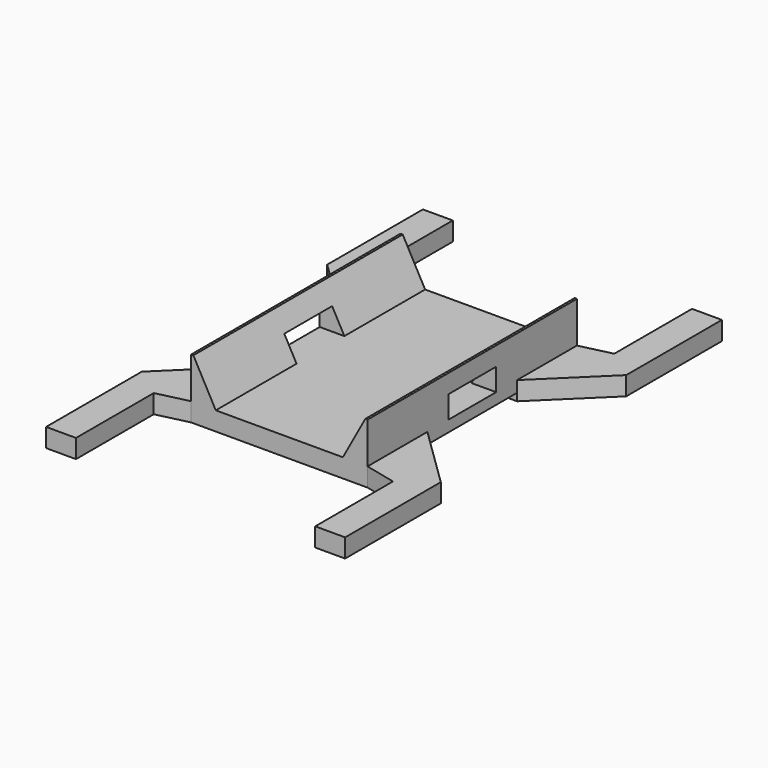
from build123d import *

# Parameters (mm, degrees)
F1_DEPTH         = 17.5
F2_W             = 8
F2_H             = 3
F2_W_2           = 15
F2_H_2           = 1
F3_DEPTH         = 50
F5_DEPTH         = 2.5
F5_COPIES2_COUNT = 2


# Not quite as in the source:
# - a pattern or mirror of a feature is missing from the dataset's text; its kind, count and spacing are read off the source's solid


with BuildPart() as f1:
    # F0 (on Front) → F1 (new body, symmetric)
    with BuildSketch(Plane.XZ):
        Polygon((-11.8, 0), (0, 0), (11.8, 0), (11.8, 8), (11.5, 8), (8.5, 2.5), (0, 2.5), (-8.5, 2.5), (-11.5, 8), (-11.8, 8), align=None)
    extrude(amount=F1_DEPTH, both=True)

    # F2 (on Right) → F3 (cut, symmetric)
    with BuildSketch(Plane.YZ):
        with Locations((0, 4)):
            Rectangle(F2_W, F2_H)
        with Locations((0, 0.5)):
            Rectangle(F2_W_2, F2_H_2)
    extrude(amount=F3_DEPTH, both=True, mode=Mode.SUBTRACT)

    # F4 (on Top) → F5 (join)
    with BuildSketch(Plane.XY):
        Polygon((16, 18.5), (11.8, 17.5), (11.8, 7.5), (20, 15.5), (20, 31.5), (16, 31.5), align=None)
    f5 = extrude(amount=F5_DEPTH)

    # F5_copies: F5 across plane
    add(f5.mirror(Plane(origin=(0, 0, 0), x_dir=(0, 0, -1), z_dir=(-1, 0, 0))))

    # F5_copies1: F5 across plane
    add(f5.mirror(Plane(origin=(0, 0, 0), x_dir=(0, 0, -1), z_dir=(0, -1, 0))))

    # F5_copies2: F5 ×2 about axis
    f5_copies2_axis = Axis((0, 0, 0), (0, 0, 1))
    for i in range(1, F5_COPIES2_COUNT):
        add(f5.rotate(f5_copies2_axis, i * 360 / F5_COPIES2_COUNT))


solid = f1.part
